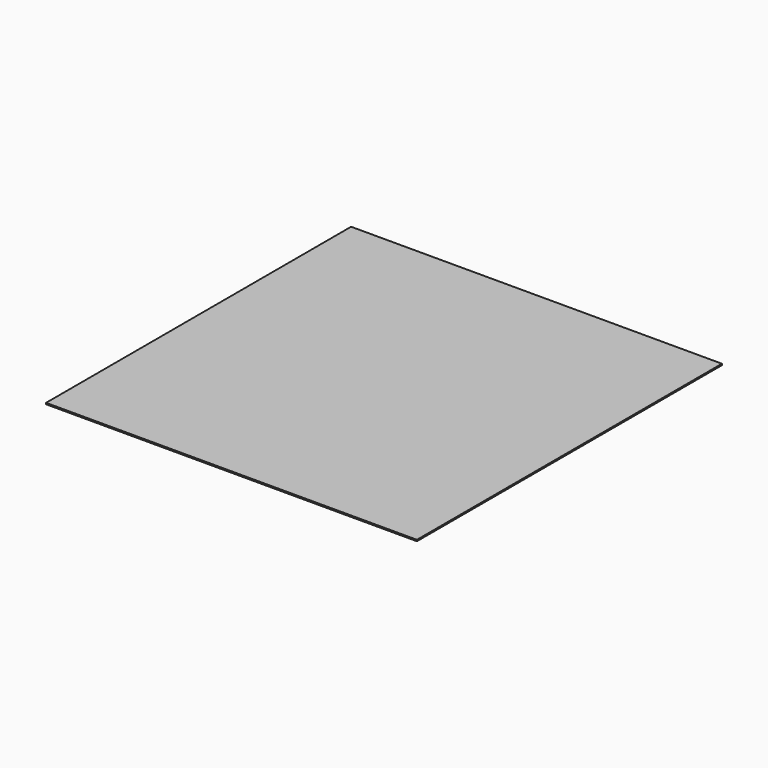
from build123d import *

# Parameters (mm, degrees)
F0_W     = 444.647287423
F0_H     = 457.2
F1_DEPTH = 1.5875


# Not quite as in the source:
# - a length typed as a fraction of an inch, garbled in the dataset ("3 / 203.2 mm" for 3/8 in), is restored


with BuildPart() as f1:
    # F0 (on Top) → F1 (new body)
    with BuildSketch(Plane.XY):
        with Locations((36.7227555253, -27.1216034889)):
            Rectangle(F0_W, F0_H)
    extrude(amount=F1_DEPTH)


solid = f1.part
